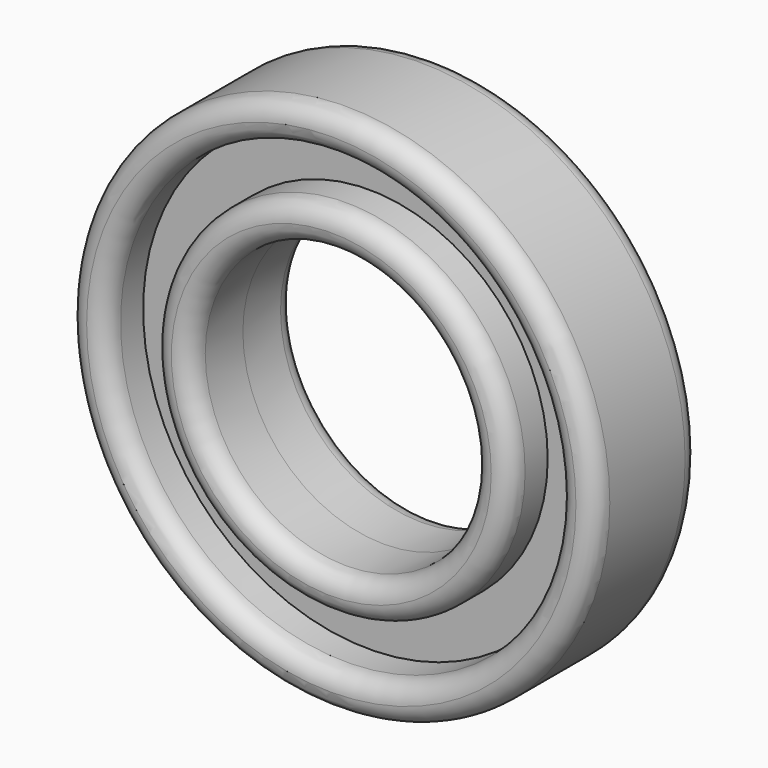
from build123d import *

# Parameters (mm, degrees)
F0_R          = 14
F0_R_2        = 12
F1_DEPTH      = 3.5
F1_DEPTH_BACK = 3.5
F2_R          = 9.5
F2_R_2        = 7.5
F3_DEPTH      = 3.5
F3_DEPTH_BACK = 3.5
F4_R          = 12.2789559666
F4_R_2        = 8.3620661584
F5_DEPTH      = 1
F5_DEPTH_BACK = 1
F6_R          = 0.99999
F6_2_R        = 0.99999


# Not quite as in the source:
# - a fillet or chamfer is up to 0.001 mm smaller than in the source, because OpenCascade refuses the exact size


with BuildPart() as f1:
    # F0 (on Front) → F1 (new body, two sides)
    with BuildSketch(Plane.XZ) as f1_sk:
        Circle(F0_R)
        Circle(F0_R_2, mode=Mode.SUBTRACT)
    extrude(amount=F1_DEPTH)
    extrude(f1_sk.sketch, amount=-F1_DEPTH_BACK)

    # F6 (radius 1 in the source; OpenCascade refuses exactly that, so slightly less here)
    f6_edges = [f1.edges().sort_by_distance(p)[0] for p in [
        (-12, -3.5, 0),
        (-14, -3.5, 0),
        (-12, 3.5, 0),
        (-14, 3.5, 0),
    ]]
    fillet(f6_edges, radius=F6_R)


with BuildPart() as f3:
    # F2 (on Front) → F3 (new body, two sides)
    with BuildSketch(Plane.XZ) as f3_sk:
        Circle(F2_R)
        Circle(F2_R_2, mode=Mode.SUBTRACT)
    extrude(amount=F3_DEPTH)
    extrude(f3_sk.sketch, amount=-F3_DEPTH_BACK)

    # F6#2 (radius 1 in the source; OpenCascade refuses exactly that, so slightly less here)
    f6_2_edges = [f3.edges().sort_by_distance(p)[0] for p in [
        (-9.5, -3.5, 0),
        (-7.5, -3.5, 0),
        (-7.5, 3.5, 0),
        (-9.5, 3.5, 0),
    ]]
    fillet(f6_2_edges, radius=F6_2_R)


with BuildPart() as f5:
    # F4 (on Front) → F5 (new body, two sides)
    with BuildSketch(Plane.XZ) as f5_sk:
        Circle(F4_R)
        Circle(F4_R_2, mode=Mode.SUBTRACT)
    extrude(amount=F5_DEPTH)
    extrude(f5_sk.sketch, amount=-F5_DEPTH_BACK)


solid = Compound([f1.part, f3.part, f5.part])
